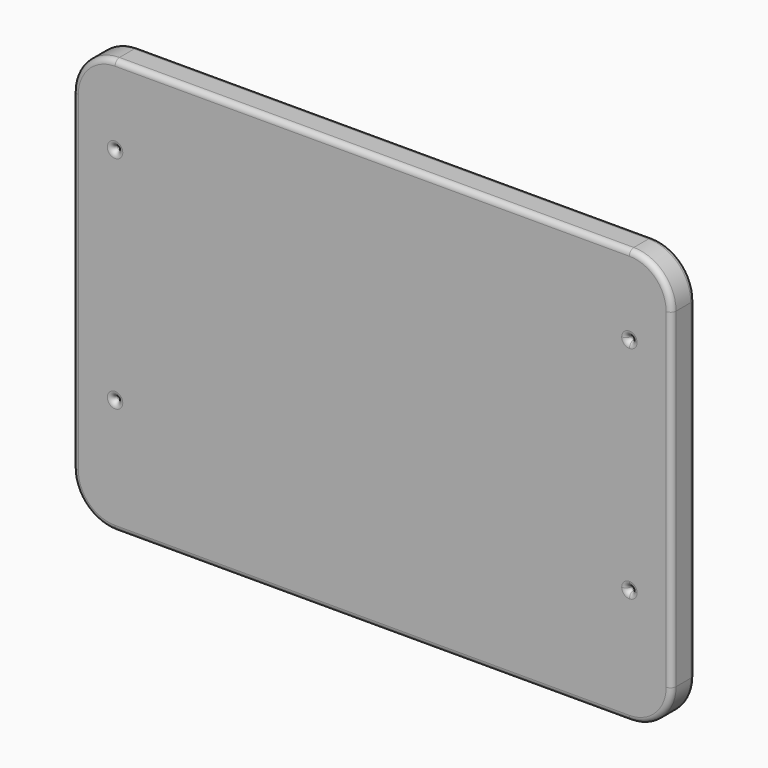
from build123d import *

# Parameters (mm, degrees)
F0_R     = 1.524
F1_DEPTH = 10.16
F2_R     = 3.81


with BuildPart() as f1:
    # F0 (on Front) → F1 (new body, symmetric)
    with BuildSketch(Plane.XZ):
        with BuildLine():
            ThreePointArc((-225.841224, 134.762077), (-246.495813, 126.206666), (-255.051224, 105.552077))
            Line((-255.051224, 105.552077), (-255.051224, -123.047923))
            ThreePointArc((-255.051224, -123.047923), (-246.495813, -143.702512), (-225.841224, -152.257923))
            Line((-225.841224, -152.257923), (129.758776, -152.257923))
            ThreePointArc((129.758776, -152.257923), (150.413365, -143.702512), (158.968776, -123.047923))
            Line((158.968776, -123.047923), (158.968776, 105.552077))
            ThreePointArc((158.968776, 105.552077), (150.413365, 126.206666), (129.758776, 134.762077))
            Line((129.758776, 134.762077), (-225.841224, 134.762077))
        make_face()
        with Locations((-225.841224, -72.247923)):
            Circle(F0_R, mode=Mode.SUBTRACT)
        with BuildLine():
            ThreePointArc((131.282776, -72.247923), (130.836407, -73.325553), (129.758776, -73.771923))
            ThreePointArc((129.758776, -73.771923), (128.681145, -73.325553), (128.234776, -72.247923))
            ThreePointArc((128.234776, -72.247923), (128.681145, -71.170292), (129.758776, -70.723923))
            ThreePointArc((129.758776, -70.723923), (130.836407, -71.170292), (131.282776, -72.247923))
        make_face(mode=Mode.SUBTRACT)
        with Locations((-225.841224, 80.152077)):
            Circle(F0_R, mode=Mode.SUBTRACT)
        with BuildLine():
            ThreePointArc((131.282776, 80.152077), (130.836407, 79.074447), (129.758776, 78.628077))
            ThreePointArc((129.758776, 78.628077), (128.681145, 79.074447), (128.234776, 80.152077))
            ThreePointArc((128.234776, 80.152077), (129.758776, 81.676077), (131.282776, 80.152077))
        make_face(mode=Mode.SUBTRACT)
    extrude(amount=F1_DEPTH, both=True)

    # F2
    f2_edges = [f1.edges().sort_by_distance(p)[0] for p in [
        (-246.495813, -10.16, 126.206666),
        (-255.051224, -10.16, -8.747923),
        (-246.495813, -10.16, -143.702512),
        (-48.041224, -10.16, -152.257923),
        (150.413365, -10.16, -143.702512),
        (158.968776, -10.16, -8.747923),
        (150.413365, -10.16, 126.206666),
        (-48.041224, -10.16, 134.762077),
        (-227.365224, -10.16, -72.247923),
        (130.836407, -10.16, -73.325553),
        (128.681145, -10.16, -73.325553),
        (128.681145, -10.16, -71.170292),
        (130.836407, -10.16, -71.170292),
        (-227.365224, -10.16, 80.152077),
        (130.836407, -10.16, 79.074447),
        (128.681145, -10.16, 79.074447),
        (129.758776, -10.16, 81.676077),
        (-246.495813, 10.16, 126.206666),
        (-255.051224, 10.16, -8.747923),
        (-246.495813, 10.16, -143.702512),
        (-48.041224, 10.16, -152.257923),
        (150.413365, 10.16, -143.702512),
        (158.968776, 10.16, -8.747923),
        (150.413365, 10.16, 126.206666),
        (-48.041224, 10.16, 134.762077),
        (-227.365224, 10.16, -72.247923),
        (130.836407, 10.16, -73.325553),
        (128.681145, 10.16, -73.325553),
        (128.681145, 10.16, -71.170292),
        (130.836407, 10.16, -71.170292),
        (-227.365224, 10.16, 80.152077),
        (130.836407, 10.16, 79.074447),
        (128.681145, 10.16, 79.074447),
        (129.758776, 10.16, 81.676077),
    ]]
    fillet(f2_edges, radius=F2_R)


solid = f1.part
